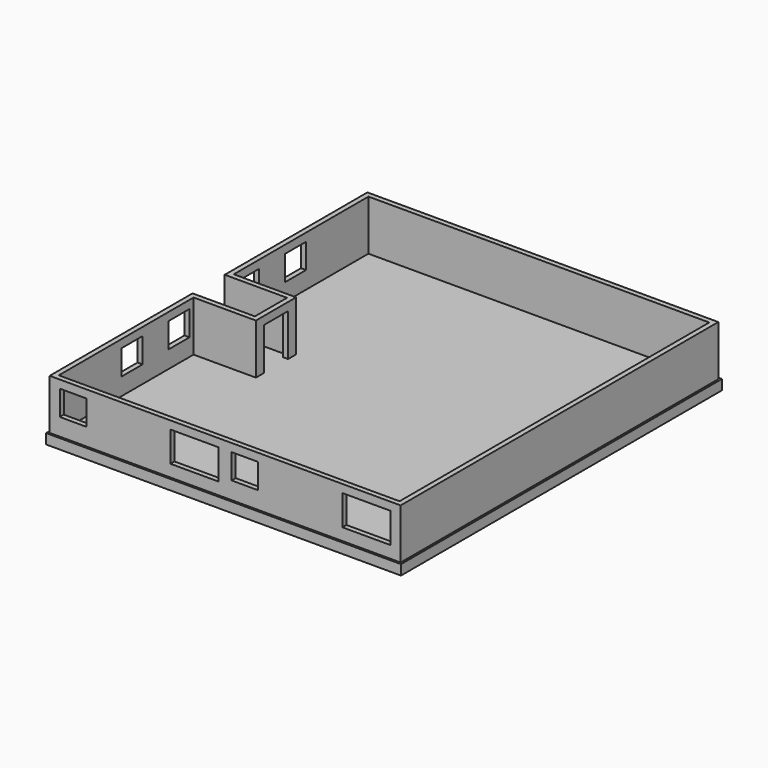
from build123d import *

# Parameters (mm, degrees)
F0_W     = 176.5
F0_H     = 199.5
F1_DEPTH = 5
F2_W     = 2.5
F2_H     = 83.7
F2_H_2   = 83.8
F3_DEPTH = 25
F4_W     = 15
F4_H     = 21
F5_DEPTH = 2.5
F6_W     = 13.2
F6_H     = 12.4
F7_DEPTH = 2.5
F8_W     = 13.2
F8_H     = 12.4
F8_W_2   = 24
F8_H_2   = 15
F9_DEPTH = 2.5


# Not quite as in the source:
# - a feature names something its author has since deleted; it is built from what else it names


with BuildPart() as f1:
    # F0 (on Top) → F1 (new body)
    with BuildSketch(Plane.XY):
        with Locations((-57.1313334405, 21.2478748113)):
            Rectangle(F0_W, F0_H)
    extrude(amount=F1_DEPTH)

    # F2 (on face) → F3 (join)
    with BuildSketch(Plane.XY.offset(5)):
        Polygon((-141.8813334405, 33.7978748113), (-144.3813334405, 33.7978748113), (-144.3813334405, 31.2978748113), (-113.3813334405, 31.2978748113), (-113.3813334405, 11.2978748113), (-144.3813334405, 11.2978748113), (-144.3813334405, 8.7978748113), (-141.8813334405, 8.7978748113), (-110.8813334405, 8.7978748113), (-110.8813334405, 33.7978748113), align=None)
        with Locations((-143.1313334405, 75.6478748113)):
            Rectangle(F2_W, F2_H)
        Polygon((30.1186665595, 119.9978748113), (-144.3813334405, 119.9978748113), (-144.3813334405, 117.4978748113), (-141.8813334405, 117.4978748113), (27.6186665595, 117.4978748113), (27.6186665595, -75.0021251887), (-141.8813334405, -75.0021251887), (-144.3813334405, -75.0021251887), (-144.3813334405, -77.5021251887), (30.1186665595, -77.5021251887), align=None)
        with Locations((-143.1313334405, -33.1021251887)):
            Rectangle(F2_W, F2_H_2)
    extrude(amount=F3_DEPTH)

    # F4 (on face) → F5 (cut, through all)
    with BuildSketch(Plane(origin=(-113.3813334405, 0, 0), x_dir=(0, -1, 0), z_dir=(-1, 0, 0))):
        with Locations((-21.2978748113, 15.5)):
            Rectangle(F4_W, F4_H)
    extrude(amount=-F5_DEPTH, mode=Mode.SUBTRACT)

    # F6 (on face) → F7 (cut, through all)
    with BuildSketch(Plane(origin=(-144.3813334405, 0, 0), x_dir=(0, -1, 0), z_dir=(-1, 0, 0))):
        with Locations((-72.0978748113, 19.8)):
            Rectangle(F6_W, F6_H)
        with Locations((-42.8978748113, 19.8)):
            Rectangle(F6_W, F6_H)
        with Locations((0.3021251887, 19.8)):
            Rectangle(F6_W, F6_H)
        with Locations((29.5021251887, 19.8)):
            Rectangle(F6_W, F6_H)
    extrude(amount=-F7_DEPTH, mode=Mode.SUBTRACT)

    # F8 (on face) → F9 (cut, through all)
    with BuildSketch(Plane.XZ.offset(77.5021251887)):
        with Locations((-132.7813334405, 19.8)):
            Rectangle(F8_W, F8_H)
        with Locations((-72.3813334405, 18.5)):
            Rectangle(F8_W_2, F8_H_2)
        with Locations((-47.2813334405, 19.8)):
            Rectangle(F8_W, F8_H)
        with Locations((13.1186665595, 18.5)):
            Rectangle(F8_W_2, F8_H_2)
    extrude(amount=-F9_DEPTH, mode=Mode.SUBTRACT)


solid = f1.part
